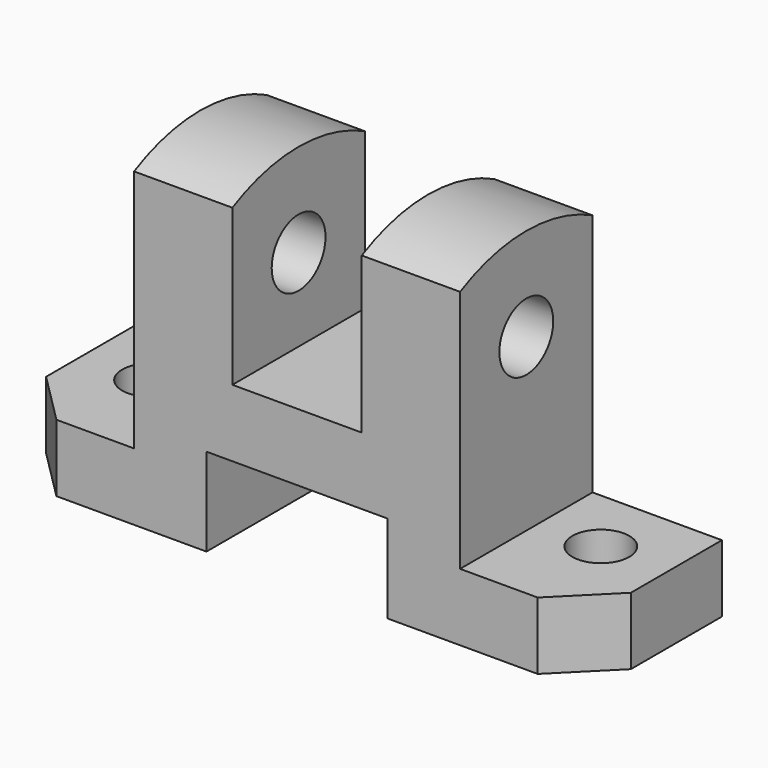
from build123d import *

# Parameters (mm, degrees)
F1_DEPTH = 16
F3_DEPTH = 19
F4_DEPTH = 88.001
F5_SIZE  = 10
F6_R     = 5.5
F7_DEPTH = 13.001


# Not quite as in the source:
# - a pattern or mirror of a feature is missing from the dataset's text; its kind, count and spacing are read off the source's solid


with BuildPart() as f1:
    # F0 (on Front) → F1 (new body, symmetric)
    with BuildSketch(Plane.XZ):
        Polygon((-56.5, 13), (-56.5, 0), (-17.5, 0), (-17.5, 17), (0, 17), (17.5, 17), (17.5, 0), (56.5, 0), (56.5, 13), (31.5, 13), (31.5, 46), (12.5, 46), (12.5, 30), (0, 30), (-12.5, 30), (-12.5, 46), (-31.5, 46), (-31.5, 13), align=None)
    extrude(amount=F1_DEPTH, both=True)

    # F2 (on face) → F3 (join)
    with BuildSketch(Plane.YZ.offset(31.5)):
        with BuildLine():
            ThreePointArc((-6.5, 46), (0, 39.5), (6.5, 46))
            ThreePointArc((6.5, 46), (0, 52.5), (-6.5, 46))
        make_face()
        with BuildLine():
            ThreePointArc((-6.5, 46), (0, 52.5), (6.5, 46))
            Line((6.5, 46), (16, 46))
            Line((16, 46), (16, 60.1287648325))
            ThreePointArc((16, 60.1287648325), (0, 64), (-16, 60.1287648325))
            Line((-16, 60.1287648325), (-16, 46))
            Line((-16, 46), (-6.5, 46))
        make_face()
    f3 = extrude(amount=-F3_DEPTH)

    # F3_copies: F3 across plane
    add(f3.mirror(Plane(origin=(0, 0, 0), x_dir=(0, 0, -1), z_dir=(-1, 0, 0))))

    # F2 (on face) → F4 (cut, through all)
    with BuildSketch(Plane.YZ.offset(31.5)):
        with BuildLine():
            Line((-6.5, 46), (6.5, 46))
            ThreePointArc((6.5, 46), (0, 52.5), (-6.5, 46))
        make_face()
        with BuildLine():
            ThreePointArc((-6.5, 46), (0, 39.5), (6.5, 46))
            Line((6.5, 46), (-6.5, 46))
        make_face()
    extrude(amount=-F4_DEPTH, mode=Mode.SUBTRACT)

    # F5
    f5_edges = [f1.edges().sort_by_distance(p)[0] for p in [
        (56.5, -16, 6.5),
        (-56.5, -16, 6.5),
    ]]
    chamfer(f5_edges, length=F5_SIZE)

    # F6 (on face) → F7 (cut, through all)
    with BuildSketch(Plane.XY.offset(13)):
        with Locations((43.5, 3)):
            Circle(F6_R)
    f7 = extrude(amount=-F7_DEPTH, mode=Mode.SUBTRACT)

    # F7_copies: F7 across plane
    add(f7.mirror(Plane(origin=(0, 0, 0), x_dir=(0, 0, -1), z_dir=(-1, 0, 0))), mode=Mode.SUBTRACT)


solid = f1.part
